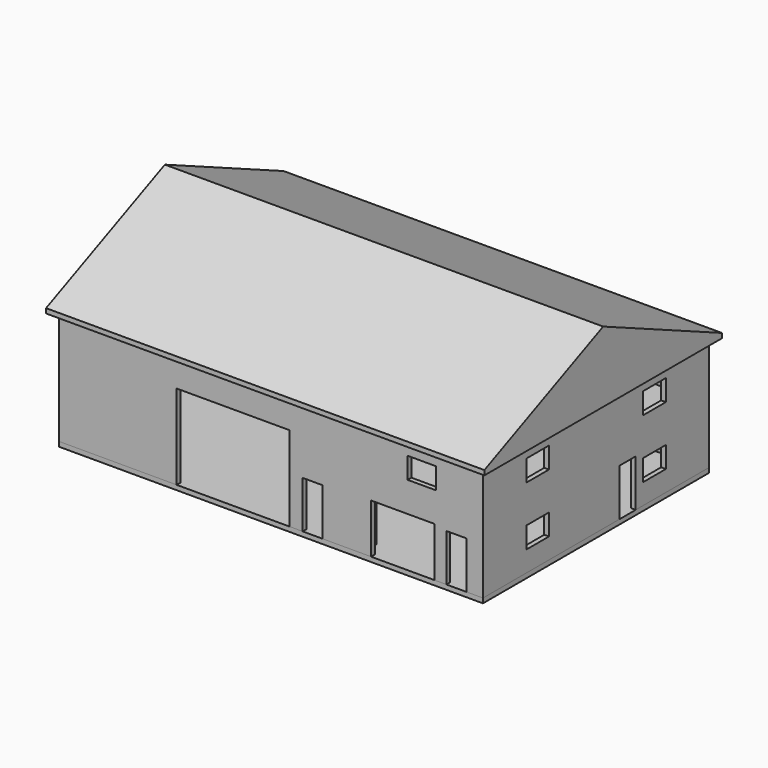
from build123d import *

# Parameters (mm, degrees)
F0_W          = 18288
F0_H          = 12192
F1_DEPTH      = 203.2
F2_W          = 18288
F2_H          = 12192
F2_W_2        = 17881.6
F2_H_2        = 11785.6
F3_DEPTH      = 4876.8
F5_DEPTH      = 9448.8
F5_DEPTH_BACK = 9448.8
F7_DEPTH      = 2336.8
F8_W          = 5181.6
F8_H          = 11785.6
F9_DEPTH      = 203.2
F10_W         = 4876.8
F10_H         = 3657.6
F10_W_2       = 863.6
F10_H_2       = 2032
F10_W_3       = 2743.2
F10_H_3       = 2133.6
F10_W_4       = 1219.2
F10_H_4       = 914.4
F11_DEPTH     = 203.2
F12_W         = 863.6
F12_H         = 2032
F13_DEPTH     = 203.2
F15_DEPTH     = 914.4
F16_W         = 2438.4
F16_H         = 2133.6
F17_DEPTH     = 152.4
F18_W         = 152.4
F18_H         = 11785.6
F19_DEPTH     = 2336.8
F20_W         = 863.6
F20_H         = 1981.2
F20_W_2       = 2438.4
F21_DEPTH     = 152.4
F22_W         = 12700
F22_H         = 254
F23_DEPTH     = 4572
F24_W         = 9956.8
F24_H         = 254
F25_DEPTH     = 4876.8
F26_W         = 5029.2
F26_H         = 50.8
F27_DEPTH     = 609.6
F28_W         = 4114.8
F28_H         = 76.2
F29_DEPTH     = 914.4
F30_W         = 1219.2
F30_H         = 914.4
F31_DEPTH     = 203.2
F32_W         = 1219.2
F32_H         = 914.4
F33_DEPTH     = 203.2
F34_W         = 1219.2
F34_H         = 914.4
F35_DEPTH     = 203.2


with BuildPart() as f1:
    # F0 (on Top) → F1 (new body)
    with BuildSketch(Plane.XY):
        Rectangle(F0_W, F0_H)
    extrude(amount=F1_DEPTH)


with BuildPart() as f3:
    # F2 (on face) → F3 (new body)
    with BuildSketch(Plane.XY.offset(203.2)):
        Rectangle(F2_W, F2_H)
        Rectangle(F2_W_2, F2_H_2, mode=Mode.SUBTRACT)
    extrude(amount=F3_DEPTH)

    # F10 (on face) → F11 (cut, through all)
    with BuildSketch(Plane.XZ.offset(6096)):
        with Locations((-1625.6, 2032)):
            Rectangle(F10_W, F10_H)
        with Locations((1803.4, 1219.2)):
            Rectangle(F10_W_2, F10_H_2)
        with Locations((5689.6, 1270)):
            Rectangle(F10_W_3, F10_H_3)
        with Locations((8001, 1219.2)):
            Rectangle(F10_W_2, F10_H_2)
        with Locations((6502.4, 4089.4)):
            Rectangle(F10_W_4, F10_H_4)
    extrude(amount=-F11_DEPTH, mode=Mode.SUBTRACT)

    # F12 (on face) → F13 (cut, through all)
    with BuildSketch(Plane.YZ.offset(9144)):
        with Locations((1701.8, 1219.2)):
            Rectangle(F12_W, F12_H)
    extrude(amount=-F13_DEPTH, mode=Mode.SUBTRACT)

    # F30 (on face) → F31 (cut, through all)
    with BuildSketch(Plane(origin=(0, 6096, 0), x_dir=(-1, 0, 0), z_dir=(0, 1, 0))):
        with Locations((-6502.4, 4089.4)):
            Rectangle(F30_W, F30_H)
        with Locations((-6502.4, 1549.4)):
            Rectangle(F30_W, F30_H)
        with Locations((-1016, 1549.4)):
            Rectangle(F30_W, F30_H)
        with Locations((6197.6, 1549.4)):
            Rectangle(F30_W, F30_H)
    extrude(amount=-F31_DEPTH, mode=Mode.SUBTRACT)

    # F32 (on face) → F33 (cut, through all)
    with BuildSketch(Plane(origin=(-9144, 0, 0), x_dir=(0, -1, 0), z_dir=(-1, 0, 0))):
        with Locations((-3149.6, 1549.4)):
            Rectangle(F32_W, F32_H)
        with Locations((3149.6, 1549.4)):
            Rectangle(F32_W, F32_H)
    extrude(amount=-F33_DEPTH, mode=Mode.SUBTRACT)

    # F34 (on face) → F35 (cut, through all)
    with BuildSketch(Plane.YZ.offset(9144)):
        with Locations((-3149.6, 1549.4)):
            Rectangle(F34_W, F34_H)
        with Locations((3149.6, 1549.4)):
            Rectangle(F34_W, F34_H)
        with Locations((-3149.6, 4089.4)):
            Rectangle(F34_W, F34_H)
        with Locations((3149.6, 4089.4)):
            Rectangle(F34_W, F34_H)
    extrude(amount=-F35_DEPTH, mode=Mode.SUBTRACT)


with BuildPart() as f5:
    # F4 (on Right) → F5 (new body, two sides)
    with BuildSketch(Plane.YZ) as f5_sk:
        Polygon((-6400.8, 5080), (6400.8, 5080), (6400.8, 5283.2), (0, 8128), (-6400.8, 5283.2), align=None)
    extrude(amount=F5_DEPTH)
    extrude(f5_sk.sketch, amount=-F5_DEPTH_BACK)


with BuildPart() as f7:
    # F6 (on face) → F7 (new body)
    with BuildSketch(Plane.XY.offset(203.2)):
        Polygon((3759.2, 5892.8), (3759.2, -5892.8), (3911.6, -5892.8), (3911.6, 203.2), (8940.8, 203.2), (8940.8, 355.6), (3911.6, 355.6), (3911.6, 5892.8), align=None)
    extrude(amount=F7_DEPTH)

    # F16 (on face) → F17 (cut, through all)
    with BuildSketch(Plane(origin=(3759.2, 0, 0), x_dir=(0, -1, 0), z_dir=(-1, 0, 0))):
        with Locations((-4368.8, 1270)):
            Rectangle(F16_W, F16_H)
        with Locations((4064, 1270)):
            Rectangle(F16_W, F16_H)
    extrude(amount=-F17_DEPTH, mode=Mode.SUBTRACT)

    # F26 (on face) → F27 (join)
    with BuildSketch(Plane(origin=(0, 355.6, 0), x_dir=(-1, 0, 0), z_dir=(0, 1, 0))):
        with Locations((-6426.2, 1854.2)):
            Rectangle(F26_W, F26_H)
        with Locations((-6426.2, 1295.4)):
            Rectangle(F26_W, F26_H)
        with Locations((-6426.2, 736.6)):
            Rectangle(F26_W, F26_H)
    extrude(amount=F27_DEPTH)

    # F28 (on face) → F29 (join)
    with BuildSketch(Plane.XZ.offset(-203.2)):
        with Locations((6883.4, 1079.5)):
            Rectangle(F28_W, F28_H)
    extrude(amount=F29_DEPTH)


with BuildPart() as f9:
    # F8 (on face) → F9 (new body)
    with BuildSketch(Plane.XY.offset(2540)):
        with Locations((6350, 0)):
            Rectangle(F8_W, F8_H)
    extrude(amount=F9_DEPTH)


with BuildPart() as f15:
    # F14 (on face) → F15 (new body)
    with BuildSketch(Plane(origin=(3759.2, 0, 0), x_dir=(0, -1, 0), z_dir=(-1, 0, 0))):
        Polygon((-371.5363917484, 2540), (1965.2636082516, 203.2), (2540, 203.2), (0, 2743.2), (-574.7363917484, 2743.2), (-1219.2, 2743.2), (-1219.2, 2540), align=None)
    extrude(amount=F15_DEPTH)


with BuildPart() as f19:
    # F18 (on face) → F19 (new body, through all)
    with BuildSketch(Plane.XY.offset(2743.2)):
        with Locations((3835.4, 0)):
            Rectangle(F18_W, F18_H)
    extrude(amount=F19_DEPTH)

    # F20 (on face) → F21 (cut, through all)
    with BuildSketch(Plane(origin=(3759.2, 0, 0), x_dir=(0, -1, 0), z_dir=(-1, 0, 0))):
        with Locations((-787.4, 3733.8)):
            Rectangle(F20_W, F20_H)
        with Locations((4064, 3733.8)):
            Rectangle(F20_W_2, F20_H)
    extrude(amount=-F21_DEPTH, mode=Mode.SUBTRACT)


with BuildPart() as f23:
    # F22 (on face) → F23 (new body)
    with BuildSketch(Plane.XZ.offset(-5892.8)):
        with Locations((-2590.8, 2870.2)):
            Rectangle(F22_W, F22_H)
    extrude(amount=F23_DEPTH)


with BuildPart() as f25:
    # F24 (on face) → F25 (new body)
    with BuildSketch(Plane.YZ.offset(-8940.8)):
        with Locations((914.4, 3098.8)):
            Rectangle(F24_W, F24_H)
    extrude(amount=F25_DEPTH)


solid = Compound([f1.part, f3.part, f5.part, f7.part, f9.part, f15.part, f19.part, f23.part, f25.part])
